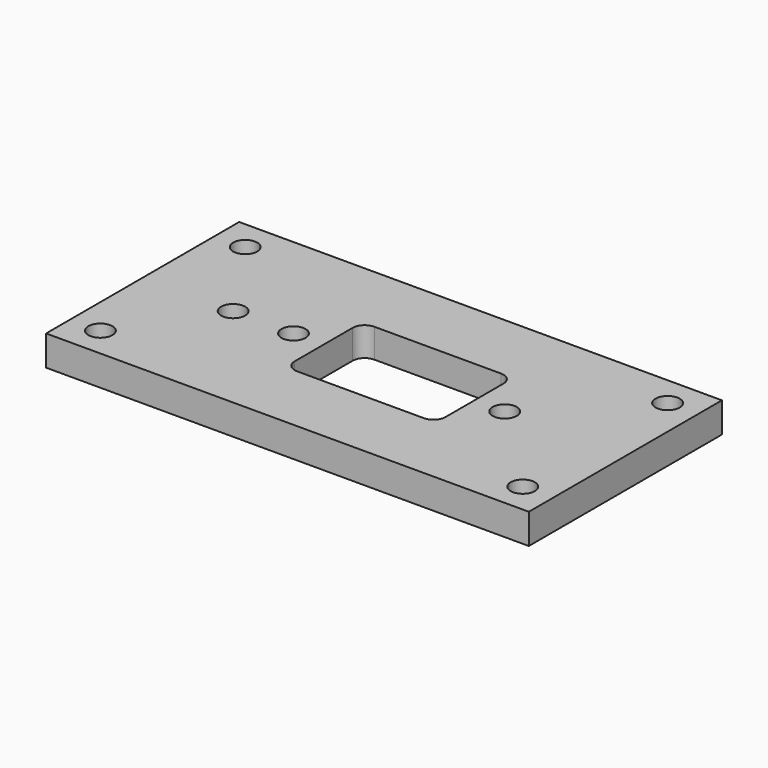
from build123d import *

# Parameters (mm, degrees)
F0_W      = 101.6
F0_H      = 50.8
F1_DEPTH  = 6.35
F3_DEPTH  = 0.254
F4_R      = 2.54
F5_DEPTH  = 6.351
F6_R      = 2.38125
F7_DEPTH  = 0.508
F8_R      = 0.79375
F9_DEPTH  = 1.27
F10_R     = 2.54
F11_DEPTH = 4.826
F13_DEPTH = 6.096


# Not quite as in the source:
# - a feature names something its author has since deleted; it is built from what else it names


with BuildPart() as f1:
    # F0 (on Top) → F1 (new body)
    with BuildSketch(Plane.XY):
        with Locations((50.8, 25.4)):
            Rectangle(F0_W, F0_H)
    extrude(amount=F1_DEPTH)

    # F2 (on face) → F3 (cut)
    with BuildSketch(Plane(origin=(0, 0, 0), x_dir=(1, 0, 0), z_dir=(0, 0, -1))):
        with BuildLine():
            Line((11.43, -14.605), (11.43, -11.43))
            Line((11.43, -11.43), (14.605, -11.43))
            ThreePointArc((14.605, -11.43), (9.1849359697, -9.1849359697), (11.43, -14.605))
        make_face()
        with BuildLine():
            Line((14.605, -11.43), (11.43, -11.43))
            Line((11.43, -11.43), (11.43, -14.605))
            ThreePointArc((11.43, -14.605), (13.6750640303, -13.6750640303), (14.605, -11.43))
        make_face()
        with BuildLine():
            Line((86.995, -11.43), (14.605, -11.43))
            ThreePointArc((14.605, -11.43), (13.6750640303, -13.6750640303), (11.43, -14.605))
            Line((11.43, -14.605), (11.43, -36.195))
            ThreePointArc((11.43, -36.195), (13.6750640303, -37.1249359697), (14.605, -39.37))
            Line((14.605, -39.37), (86.995, -39.37))
            ThreePointArc((86.995, -39.37), (87.9249359697, -37.1249359697), (90.17, -36.195))
            Line((90.17, -36.195), (90.17, -14.605))
            ThreePointArc((90.17, -14.605), (87.9249359697, -13.6750640303), (86.995, -11.43))
        make_face()
        with BuildLine():
            ThreePointArc((93.345, -11.43), (90.17, -8.255), (86.995, -11.43))
            Line((86.995, -11.43), (90.17, -11.43))
            Line((90.17, -11.43), (90.17, -14.605))
            ThreePointArc((90.17, -14.605), (92.4150640303, -13.6750640303), (93.345, -11.43))
        make_face()
        with BuildLine():
            Line((90.17, -11.43), (86.995, -11.43))
            ThreePointArc((86.995, -11.43), (87.9249359697, -13.6750640303), (90.17, -14.605))
            Line((90.17, -14.605), (90.17, -11.43))
        make_face()
        with BuildLine():
            ThreePointArc((14.605, -39.37), (13.6750640303, -37.1249359697), (11.43, -36.195))
            Line((11.43, -36.195), (11.43, -39.37))
            Line((11.43, -39.37), (14.605, -39.37))
        make_face()
        with BuildLine():
            Line((11.43, -39.37), (11.43, -36.195))
            ThreePointArc((11.43, -36.195), (9.1849359697, -41.6150640303), (14.605, -39.37))
            Line((14.605, -39.37), (11.43, -39.37))
        make_face()
        with BuildLine():
            ThreePointArc((93.345, -39.37), (92.4150640303, -37.1249359697), (90.17, -36.195))
            Line((90.17, -36.195), (90.17, -39.37))
            Line((90.17, -39.37), (86.995, -39.37))
            ThreePointArc((86.995, -39.37), (90.17, -42.545), (93.345, -39.37))
        make_face()
        with BuildLine():
            Line((90.17, -39.37), (90.17, -36.195))
            ThreePointArc((90.17, -36.195), (87.9249359697, -37.1249359697), (86.995, -39.37))
            Line((86.995, -39.37), (90.17, -39.37))
        make_face()
    extrude(amount=-F3_DEPTH, mode=Mode.SUBTRACT)

    # F4 (on face) → F5 (cut, through all)
    with BuildSketch(Plane(origin=(0, 0, 0), x_dir=(1, 0, 0), z_dir=(0, 0, -1))):
        with Locations((95.25, -6.35)):
            Circle(F4_R)
        with Locations((6.35, -6.35)):
            Circle(F4_R)
        with Locations((6.35, -44.45)):
            Circle(F4_R)
        with Locations((95.25, -44.45)):
            Circle(F4_R)
    extrude(amount=-F5_DEPTH, mode=Mode.SUBTRACT)

    # F6 (on face) → F7 (cut)
    with BuildSketch(Plane(origin=(0, 0, 0.254), x_dir=(1, 0, 0), z_dir=(0, 0, -1))):
        with Locations((31.75, -25.4)):
            Circle(F6_R)
        with Locations((19.05, -25.4)):
            Circle(F6_R)
        with Locations((76.2, -25.4)):
            Circle(F6_R)
    extrude(amount=-F7_DEPTH, mode=Mode.SUBTRACT)

    # F8 (on face) → F9 (cut)
    with BuildSketch(Plane(origin=(0, 0, 0.762), x_dir=(1, 0, 0), z_dir=(0, 0, -1))):
        with Locations((19.05, -25.4)):
            Circle(F8_R)
        with Locations((31.75, -25.4)):
            Circle(F8_R)
        with Locations((76.2, -25.4)):
            Circle(F8_R)
    extrude(amount=-F9_DEPTH, mode=Mode.SUBTRACT)

    # F10 (on face) → F11 (cut)
    with BuildSketch(Plane.XY.offset(6.35)):
        with Locations((19.05, 25.4)):
            Circle(F10_R)
        with Locations((31.75, 25.4)):
            Circle(F10_R)
        with Locations((76.2, 25.4)):
            Circle(F10_R)
    extrude(amount=-F11_DEPTH, mode=Mode.SUBTRACT)

    # F12 (on face) → F13 (cut, through all)
    with BuildSketch(Plane(origin=(0, 0, 0.254), x_dir=(1, 0, 0), z_dir=(0, 0, -1))):
        with BuildLine():
            Line((67.31, -15.24), (40.64, -15.24))
            ThreePointArc((40.64, -15.24), (38.8439487758, -15.9839487758), (38.1, -17.78))
            Line((38.1, -17.78), (38.1, -33.02))
            ThreePointArc((38.1, -33.02), (38.8439487758, -34.8160512242), (40.64, -35.56))
            Line((40.64, -35.56), (67.31, -35.56))
            ThreePointArc((67.31, -35.56), (69.1060512242, -34.8160512242), (69.85, -33.02))
            Line((69.85, -33.02), (69.85, -17.78))
            ThreePointArc((69.85, -17.78), (69.1060512242, -15.9839487758), (67.31, -15.24))
        make_face()
    extrude(amount=-F13_DEPTH, mode=Mode.SUBTRACT)


solid = f1.part
